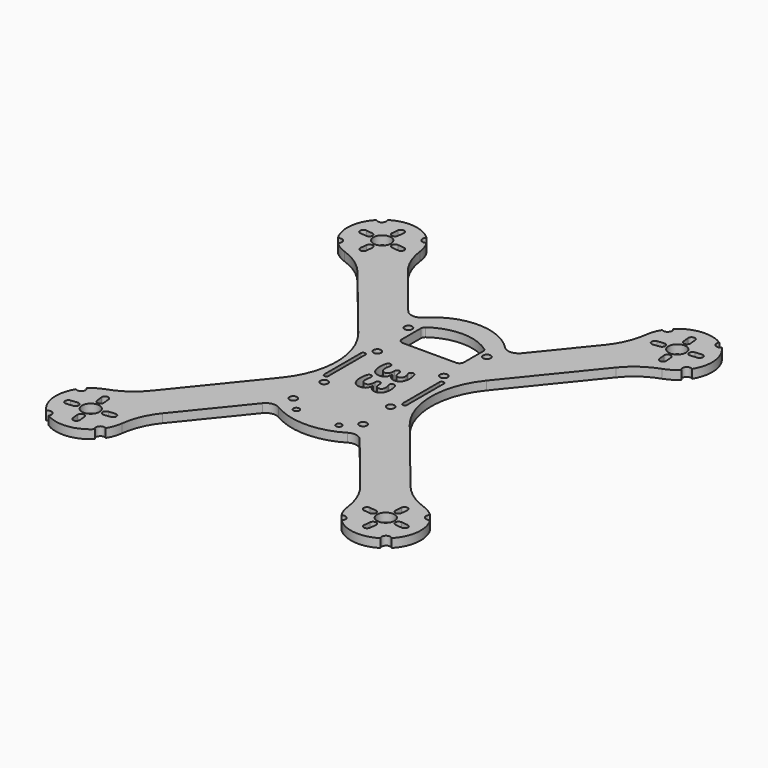
from build123d import *

# Parameters (mm, degrees)
F0_R        = 4
F0_R_2      = 1.35
F0_R_3      = 1.75
F1_DEPTH    = 4
F2_T1_DEPTH = 4


# Not quite as in the source:
# - a fillet or chamfer that OpenCascade refuses, or shapes differently, is made with other operations: its cross-section is extruded or revolved along the edge and cut away or added


with BuildPart() as f1:
    # F0 (on Top) → F1 (new body)
    with BuildSketch(Plane.XY):
        with BuildLine():
            ThreePointArc((59.2954813788, 58.9226797885), (65.4077135301, 64.6212321295), (72.8546961891, 68.4127133611))
            ThreePointArc((72.8546961891, 68.4127133611), (75.9892117021, 69.8870591003), (78.732954082, 72.0014764226))
            ThreePointArc((78.732954082, 72.0014764226), (78.5319854983, 74.7327053819), (81.2453142699, 75.1039828748))
            ThreePointArc((81.2453142699, 75.1039828748), (83.5642923637, 85.2156462689), (79.1936564719, 94.6242029008))
            ThreePointArc((79.1936564719, 94.6242029008), (76.4624275126, 94.423234317), (76.0911500197, 97.1365630887))
            ThreePointArc((76.0911500197, 97.1365630887), (65.9794866256, 99.4555411825), (56.5709299937, 95.0849052907))
            ThreePointArc((56.5709299937, 95.0849052907), (56.7718985775, 92.3536763313), (54.0585698058, 91.9823988384))
            ThreePointArc((54.0585698058, 91.9823988384), (52.5608136924, 88.8590017319), (51.7703883652, 85.4864491879))
            ThreePointArc((51.7703883652, 85.4864491879), (49.6100748513, 77.4139076937), (45.3068540726, 70.2504468274))
            Line((45.3068540726, 70.2504468274), (26.0751424851, 46.5012608726))
            ThreePointArc((26.0751424851, 46.5012608726), (22.420247462, 44.6531941399), (18.6104751491, 46.1562720492))
            ThreePointArc((18.6104751491, 46.1562720492), (0, 54), (-18.6104751491, 46.1562720492))
            ThreePointArc((-18.6104751491, 46.1562720492), (-22.420247462, 44.6531941399), (-26.0751424851, 46.5012608726))
            Line((-26.0751424851, 46.5012608726), (-45.3068540726, 70.2504468274))
            ThreePointArc((-45.3068540726, 70.2504468274), (-49.6100748513, 77.4139076937), (-51.7703883652, 85.4864491879))
            ThreePointArc((-51.7703883652, 85.4864491879), (-52.5608136924, 88.8590017319), (-54.0585698058, 91.9823988384))
            ThreePointArc((-54.0585698058, 91.9823988384), (-56.7718985775, 92.3536763313), (-56.5709299937, 95.0849052907))
            ThreePointArc((-56.5709299937, 95.0849052907), (-65.9794866256, 99.4555411825), (-76.0911500197, 97.1365630887))
            ThreePointArc((-76.0911500197, 97.1365630887), (-76.4624275126, 94.423234317), (-79.1936564719, 94.6242029008))
            ThreePointArc((-79.1936564719, 94.6242029008), (-83.5642923637, 85.2156462689), (-81.2453142699, 75.1039828748))
            ThreePointArc((-81.2453142699, 75.1039828748), (-78.5319854983, 74.7327053819), (-78.732954082, 72.0014764226))
            ThreePointArc((-78.732954082, 72.0014764226), (-75.9892117021, 69.8870591003), (-72.8546961891, 68.4127133611))
            ThreePointArc((-72.8546961891, 68.4127133611), (-65.4077135301, 64.6212321295), (-59.2954813788, 58.9226797885))
            Line((-59.2954813788, 58.9226797885), (-29.4173122483, 22.0262136867))
            ThreePointArc((-29.4173122483, 22.0262136867), (-21.6174208993, 0), (-29.4173122483, -22.0262136867))
            Line((-29.4173122483, -22.0262136867), (-59.2954813788, -58.9226797885))
            ThreePointArc((-59.2954813788, -58.9226797885), (-65.4077135301, -64.6212321295), (-72.8546961891, -68.4127133611))
            ThreePointArc((-72.8546961891, -68.4127133611), (-75.9892117021, -69.8870591003), (-78.732954082, -72.0014764226))
            ThreePointArc((-78.732954082, -72.0014764226), (-78.5319854983, -74.7327053819), (-81.2453142699, -75.1039828748))
            ThreePointArc((-81.2453142699, -75.1039828748), (-83.5642923637, -85.2156462689), (-79.1936564719, -94.6242029008))
            ThreePointArc((-79.1936564719, -94.6242029008), (-76.4624275126, -94.423234317), (-76.0911500197, -97.1365630887))
            ThreePointArc((-76.0911500197, -97.1365630887), (-65.9794866256, -99.4555411825), (-56.5709299937, -95.0849052907))
            ThreePointArc((-56.5709299937, -95.0849052907), (-56.7718985775, -92.3536763313), (-54.0585698058, -91.9823988384))
            ThreePointArc((-54.0585698058, -91.9823988384), (-52.5608136924, -88.8590017319), (-51.7703883652, -85.4864491879))
            ThreePointArc((-51.7703883652, -85.4864491879), (-49.6100748513, -77.4139076937), (-45.3068540726, -70.2504468274))
            Line((-45.3068540726, -70.2504468274), (-22.2716253028, -41.8043083194))
            ThreePointArc((-22.2716253028, -41.8043083194), (-19.2665196055, -40.0290710679), (-15.8322988989, -40.6521727365))
            ThreePointArc((-15.8322988989, -40.6521727365), (0, -45), (15.8322988989, -40.6521727365))
            ThreePointArc((15.8322988989, -40.6521727365), (19.2665196055, -40.0290710679), (22.2716253028, -41.8043083194))
            Line((22.2716253028, -41.8043083194), (45.3068540726, -70.2504468274))
            ThreePointArc((45.3068540726, -70.2504468274), (49.6100748513, -77.4139076937), (51.7703883652, -85.4864491879))
            ThreePointArc((51.7703883652, -85.4864491879), (52.5608136924, -88.8590017319), (54.0585698058, -91.9823988384))
            ThreePointArc((54.0585698058, -91.9823988384), (56.7718985775, -92.3536763313), (56.5709299937, -95.0849052907))
            ThreePointArc((56.5709299937, -95.0849052907), (65.9794866256, -99.4555411825), (76.0911500197, -97.1365630887))
            ThreePointArc((76.0911500197, -97.1365630887), (76.4624275126, -94.423234317), (79.1936564719, -94.6242029008))
            ThreePointArc((79.1936564719, -94.6242029008), (83.5642923637, -85.2156462689), (81.2453142699, -75.1039828748))
            ThreePointArc((81.2453142699, -75.1039828748), (78.5319854983, -74.7327053819), (78.732954082, -72.0014764226))
            ThreePointArc((78.732954082, -72.0014764226), (75.9892117021, -69.8870591003), (72.8546961891, -68.4127133611))
            ThreePointArc((72.8546961891, -68.4127133611), (65.4077135301, -64.6212321295), (59.2954813788, -58.9226797885))
            Line((59.2954813788, -58.9226797885), (29.4173122483, -22.0262136867))
            ThreePointArc((29.4173122483, -22.0262136867), (21.6174208993, 0), (29.4173122483, 22.0262136867))
            Line((29.4173122483, 22.0262136867), (59.2954813788, 58.9226797885))
        make_face()
        with BuildLine():
            Line((-68.1507044799, -93.1479415575), (-68.4642898697, -90.1643758714))
            ThreePointArc((-68.4642898697, -90.1643758714), (-67.1292997215, -88.5158003335), (-65.4807241836, -89.8507904816))
            Line((-65.4807241836, -89.8507904816), (-65.1671387938, -92.8343561677))
            ThreePointArc((-65.1671387938, -92.8343561677), (-66.5021289419, -94.4829317057), (-68.1507044799, -93.1479415575))
        make_face(mode=Mode.SUBTRACT)
        with BuildLine():
            Line((-77.2566927388, -83.0444284146), (-74.2731270527, -82.7308430248))
            ThreePointArc((-74.2731270527, -82.7308430248), (-72.6245515147, -84.065833173), (-73.9595416628, -85.7144087109))
            Line((-73.9595416628, -85.7144087109), (-76.943107349, -86.0279941007))
            ThreePointArc((-76.943107349, -86.0279941007), (-78.5916828869, -84.6930039526), (-77.2566927388, -83.0444284146))
        make_face(mode=Mode.SUBTRACT)
        with Locations((-67.6519420379, -83.5431908566)):
            Circle(F0_R, mode=Mode.SUBTRACT)
        with BuildLine():
            ThreePointArc((-66.839594206, -76.9220058418), (-68.1745843542, -78.5705813798), (-69.8231598921, -77.2355912316))
            Line((-69.8231598921, -77.2355912316), (-70.136745282, -74.2520255455))
            ThreePointArc((-70.136745282, -74.2520255455), (-68.8017551338, -72.6034500076), (-67.1531795958, -73.9384401557))
            Line((-67.1531795958, -73.9384401557), (-66.839594206, -76.9220058418))
        make_face(mode=Mode.SUBTRACT)
        with BuildLine():
            Line((-58.047191337, -84.0419532986), (-61.0307570231, -84.3555386884))
            ThreePointArc((-61.0307570231, -84.3555386884), (-62.679332561, -83.0205485403), (-61.3443424129, -81.3719730023))
            Line((-61.3443424129, -81.3719730023), (-58.3607767268, -81.0583876125))
            ThreePointArc((-58.3607767268, -81.0583876125), (-56.7122011888, -82.3933777607), (-58.047191337, -84.0419532986))
        make_face(mode=Mode.SUBTRACT)
        with Locations((-9.75, -38)):
            Circle(F0_R_2, mode=Mode.SUBTRACT)
        with Locations((-16, -32)):
            Circle(F0_R_3, mode=Mode.SUBTRACT)
        with Locations((-15.25, -15.25)):
            Circle(F0_R_3, mode=Mode.SUBTRACT)
        with BuildLine():
            add(Edge.make_bspline(
                [(6.2055121528, -8.4370659722), (5.33203125, -9.6857638889), (3.7764756944, -9.6857638889)],
                knots=[0, 0, 0, 1, 1, 1], degree=2))
            add(Edge.make_bspline(
                [(3.7764756944, -9.6857638889), (2.4761284722, -9.6857638889), (1.5646701389, -8.8973524306)],
                knots=[0, 0, 0, 1, 1, 1], degree=2))
            add(Edge.make_bspline(
                [(1.5646701389, -8.8973524306), (0.6532118056, -8.1089409722), (0.3098958333, -6.6840277778)],
                knots=[0, 0, 0, 1, 1, 1], degree=2))
            Line((0.3098958333, -6.6840277778), (0.2552083333, -6.6840277778))
            add(Edge.make_bspline(
                [(0.2552083333, -6.6840277778), (0.0455729167, -8.3671875), (-0.7671440972, -9.2300347222)],
                knots=[0, 0, 0, 1, 1, 1], degree=2))
            add(Edge.make_bspline(
                [(-0.7671440972, -9.2300347222), (-1.5798611111, -10.0928819444), (-2.9561631944, -10.0928819444)],
                knots=[0, 0, 0, 1, 1, 1], degree=2))
            add(Edge.make_bspline(
                [(-2.9561631944, -10.0928819444), (-4.9583333333, -10.0928819444), (-6.0748697917, -8.640625)],
                knots=[0, 0, 0, 1, 1, 1], degree=2))
            add(Edge.make_bspline(
                [(-6.0748697917, -8.640625), (-7.19140625, -7.1883680556), (-7.19140625, -4.4934895833)],
                knots=[0, 0, 0, 1, 1, 1], degree=2))
            add(Edge.make_bspline(
                [(-7.19140625, -4.4934895833), (-7.19140625, -2.2330729167), (-6.4409722222, -0.4861111111)],
                knots=[0, 0, 0, 1, 1, 1], degree=2))
            Line((-6.4409722222, -0.4861111111), (-3.9435763889, -0.4861111111))
            add(Edge.make_bspline(
                [(-3.9435763889, -0.4861111111), (-4.3506944444, -1.2912326389), (-4.607421875, -2.2604166667)],
                knots=[0, 0, 0, 1, 1, 1], degree=2))
            add(Edge.make_bspline(
                [(-4.607421875, -2.2604166667), (-4.8641493056, -3.2296006944), (-4.8641493056, -4.1775173611)],
                knots=[0, 0, 0, 1, 1, 1], degree=2))
            add(Edge.make_bspline(
                [(-4.8641493056, -4.1775173611), (-4.8641493056, -5.6328125), (-4.3704427083, -6.3255208333)],
                knots=[0, 0, 0, 1, 1, 1], degree=2))
            add(Edge.make_bspline(
                [(-4.3704427083, -6.3255208333), (-3.8767361111, -7.0182291667), (-2.7829861111, -7.0182291667)],
                knots=[0, 0, 0, 1, 1, 1], degree=2))
            add(Edge.make_bspline(
                [(-2.7829861111, -7.0182291667), (-1.8077256944, -7.0182291667), (-1.3990885417, -6.220703125)],
                knots=[0, 0, 0, 1, 1, 1], degree=2))
            add(Edge.make_bspline(
                [(-1.3990885417, -6.220703125), (-0.9904513889, -5.4231770833), (-0.9904513889, -3.6762152778)],
                knots=[0, 0, 0, 1, 1, 1], degree=2))
            Line((-0.9904513889, -3.6762152778), (-0.9904513889, -2.6219618056))
            Line((-0.9904513889, -2.6219618056), (1.2608506944, -2.6219618056))
            Line((1.2608506944, -2.6219618056), (1.2608506944, -3.6944444444))
            add(Edge.make_bspline(
                [(1.2608506944, -3.6944444444), (1.2608506944, -5.3077256944), (1.6831597222, -6.0536024306)],
                knots=[0, 0, 0, 1, 1, 1], degree=2))
            add(Edge.make_bspline(
                [(1.6831597222, -6.0536024306), (2.10546875, -6.7994791667), (3.1293402778, -6.7994791667)],
                knots=[0, 0, 0, 1, 1, 1], degree=2))
            add(Edge.make_bspline(
                [(3.1293402778, -6.7994791667), (4.7061631944, -6.7994791667), (4.7061631944, -4.8246527778)],
                knots=[0, 0, 0, 1, 1, 1], degree=2))
            add(Edge.make_bspline(
                [(4.7061631944, -4.8246527778), (4.7061631944, -4.1410590278), (4.4782986111, -3.4331597222)],
                knots=[0, 0, 0, 1, 1, 1], degree=2))
            add(Edge.make_bspline(
                [(4.4782986111, -3.4331597222), (4.2504340278, -2.7252604167), (3.69140625, -1.8624131944)],
                knots=[0, 0, 0, 1, 1, 1], degree=2))
            Line((3.69140625, -1.8624131944), (5.7118055556, -0.5043402778))
            add(Edge.make_bspline(
                [(5.7118055556, -0.5043402778), (7.0789930556, -2.4032118056), (7.0789930556, -5.0342881944)],
                knots=[0, 0, 0, 1, 1, 1], degree=2))
            add(Edge.make_bspline(
                [(7.0789930556, -5.0342881944), (7.0789930556, -7.1883680556), (6.2055121528, -8.4370659722)],
                knots=[0, 0, 0, 1, 1, 1], degree=2))
        make_face(mode=Mode.SUBTRACT)
        with BuildLine():
            ThreePointArc((61.3443424129, -81.3719730023), (62.679332561, -83.0205485403), (61.0307570231, -84.3555386884))
            Line((61.0307570231, -84.3555386884), (58.047191337, -84.0419532986))
            ThreePointArc((58.047191337, -84.0419532986), (56.7122011888, -82.3933777607), (58.3607767268, -81.0583876125))
            Line((58.3607767268, -81.0583876125), (61.3443424129, -81.3719730023))
        make_face(mode=Mode.SUBTRACT)
        with BuildLine():
            ThreePointArc((65.4807241836, -89.8507904816), (67.1292997215, -88.5158003335), (68.4642898697, -90.1643758714))
            Line((68.4642898697, -90.1643758714), (68.1507044799, -93.1479415575))
            ThreePointArc((68.1507044799, -93.1479415575), (66.5021289419, -94.4829317057), (65.1671387938, -92.8343561677))
            Line((65.1671387938, -92.8343561677), (65.4807241836, -89.8507904816))
        make_face(mode=Mode.SUBTRACT)
        with Locations((67.6519420379, -83.5431908566)):
            Circle(F0_R, mode=Mode.SUBTRACT)
        with BuildLine():
            ThreePointArc((69.8231598921, -77.2355912316), (68.1745843542, -78.5705813798), (66.839594206, -76.9220058418))
            Line((66.839594206, -76.9220058418), (67.1531795958, -73.9384401557))
            ThreePointArc((67.1531795958, -73.9384401557), (68.8017551338, -72.6034500076), (70.136745282, -74.2520255455))
            Line((70.136745282, -74.2520255455), (69.8231598921, -77.2355912316))
        make_face(mode=Mode.SUBTRACT)
        with BuildLine():
            ThreePointArc((73.9595416628, -85.7144087109), (72.6245515147, -84.065833173), (74.2731270527, -82.7308430248))
            Line((74.2731270527, -82.7308430248), (77.2566927388, -83.0444284146))
            ThreePointArc((77.2566927388, -83.0444284146), (78.5916828869, -84.6930039526), (76.943107349, -86.0279941007))
            Line((76.943107349, -86.0279941007), (73.9595416628, -85.7144087109))
        make_face(mode=Mode.SUBTRACT)
        with Locations((9.75, -38)):
            Circle(F0_R_2, mode=Mode.SUBTRACT)
        with Locations((16, -32)):
            Circle(F0_R_3, mode=Mode.SUBTRACT)
        with Locations((15.25, -15.25)):
            Circle(F0_R_3, mode=Mode.SUBTRACT)
        with BuildLine():
            Line((-19, -10.5), (-19, 10.5))
            ThreePointArc((-19, 10.5), (-18, 11.5), (-17, 10.5))
            Line((-17, 10.5), (-17, -10.5))
            ThreePointArc((-17, -10.5), (-18, -11.5), (-19, -10.5))
        make_face(mode=Mode.SUBTRACT)
        with BuildLine():
            add(Edge.make_bspline(
                [(6.2055121528, 2.6614583333), (5.33203125, 1.4127604167), (3.7764756944, 1.4127604167)],
                knots=[0, 0, 0, 1, 1, 1], degree=2))
            add(Edge.make_bspline(
                [(3.7764756944, 1.4127604167), (2.4761284722, 1.4127604167), (1.5646701389, 2.201171875)],
                knots=[0, 0, 0, 1, 1, 1], degree=2))
            add(Edge.make_bspline(
                [(1.5646701389, 2.201171875), (0.6532118056, 2.9895833333), (0.3098958333, 4.4144965278)],
                knots=[0, 0, 0, 1, 1, 1], degree=2))
            Line((0.3098958333, 4.4144965278), (0.2552083333, 4.4144965278))
            add(Edge.make_bspline(
                [(0.2552083333, 4.4144965278), (0.0455729167, 2.7313368056), (-0.7671440972, 1.8684895833)],
                knots=[0, 0, 0, 1, 1, 1], degree=2))
            add(Edge.make_bspline(
                [(-0.7671440972, 1.8684895833), (-1.5798611111, 1.0056423611), (-2.9561631944, 1.0056423611)],
                knots=[0, 0, 0, 1, 1, 1], degree=2))
            add(Edge.make_bspline(
                [(-2.9561631944, 1.0056423611), (-4.9583333333, 1.0056423611), (-6.0748697917, 2.4578993056)],
                knots=[0, 0, 0, 1, 1, 1], degree=2))
            add(Edge.make_bspline(
                [(-6.0748697917, 2.4578993056), (-7.19140625, 3.91015625), (-7.19140625, 6.6050347222)],
                knots=[0, 0, 0, 1, 1, 1], degree=2))
            add(Edge.make_bspline(
                [(-7.19140625, 6.6050347222), (-7.19140625, 8.8654513889), (-6.4409722222, 10.6124131944)],
                knots=[0, 0, 0, 1, 1, 1], degree=2))
            Line((-6.4409722222, 10.6124131944), (-3.9435763889, 10.6124131944))
            add(Edge.make_bspline(
                [(-3.9435763889, 10.6124131944), (-4.3506944444, 9.8072916667), (-4.607421875, 8.8381076389)],
                knots=[0, 0, 0, 1, 1, 1], degree=2))
            add(Edge.make_bspline(
                [(-4.607421875, 8.8381076389), (-4.8641493056, 7.8689236111), (-4.8641493056, 6.9210069444)],
                knots=[0, 0, 0, 1, 1, 1], degree=2))
            add(Edge.make_bspline(
                [(-4.8641493056, 6.9210069444), (-4.8641493056, 5.4657118056), (-4.3704427083, 4.7730034722)],
                knots=[0, 0, 0, 1, 1, 1], degree=2))
            add(Edge.make_bspline(
                [(-4.3704427083, 4.7730034722), (-3.8767361111, 4.0802951389), (-2.7829861111, 4.0802951389)],
                knots=[0, 0, 0, 1, 1, 1], degree=2))
            add(Edge.make_bspline(
                [(-2.7829861111, 4.0802951389), (-1.8077256944, 4.0802951389), (-1.3990885417, 4.8778211806)],
                knots=[0, 0, 0, 1, 1, 1], degree=2))
            add(Edge.make_bspline(
                [(-1.3990885417, 4.8778211806), (-0.9904513889, 5.6753472222), (-0.9904513889, 7.4223090278)],
                knots=[0, 0, 0, 1, 1, 1], degree=2))
            Line((-0.9904513889, 7.4223090278), (-0.9904513889, 8.4765625))
            Line((-0.9904513889, 8.4765625), (1.2608506944, 8.4765625))
            Line((1.2608506944, 8.4765625), (1.2608506944, 7.4040798611))
            add(Edge.make_bspline(
                [(1.2608506944, 7.4040798611), (1.2608506944, 5.7907986111), (1.6831597222, 5.044921875)],
                knots=[0, 0, 0, 1, 1, 1], degree=2))
            add(Edge.make_bspline(
                [(1.6831597222, 5.044921875), (2.10546875, 4.2990451389), (3.1293402778, 4.2990451389)],
                knots=[0, 0, 0, 1, 1, 1], degree=2))
            add(Edge.make_bspline(
                [(3.1293402778, 4.2990451389), (4.7061631944, 4.2990451389), (4.7061631944, 6.2738715278)],
                knots=[0, 0, 0, 1, 1, 1], degree=2))
            add(Edge.make_bspline(
                [(4.7061631944, 6.2738715278), (4.7061631944, 6.9574652778), (4.4782986111, 7.6653645833)],
                knots=[0, 0, 0, 1, 1, 1], degree=2))
            add(Edge.make_bspline(
                [(4.4782986111, 7.6653645833), (4.2504340278, 8.3732638889), (3.69140625, 9.2361111111)],
                knots=[0, 0, 0, 1, 1, 1], degree=2))
            Line((3.69140625, 9.2361111111), (5.7118055556, 10.5941840278))
            add(Edge.make_bspline(
                [(5.7118055556, 10.5941840278), (7.0789930556, 8.6953125), (7.0789930556, 6.0642361111)],
                knots=[0, 0, 0, 1, 1, 1], degree=2))
            add(Edge.make_bspline(
                [(7.0789930556, 6.0642361111), (7.0789930556, 3.91015625), (6.2055121528, 2.6614583333)],
                knots=[0, 0, 0, 1, 1, 1], degree=2))
        make_face(mode=Mode.SUBTRACT)
        with Locations((-15.25, 15.25)):
            Circle(F0_R_3, mode=Mode.SUBTRACT)
        with Locations((-18, 36.5)):
            Circle(F0_R_3, mode=Mode.SUBTRACT)
        with BuildLine():
            ThreePointArc((-73.9595416628, 85.7144087109), (-72.6245515147, 84.065833173), (-74.2731270527, 82.7308430248))
            Line((-74.2731270527, 82.7308430248), (-77.2566927388, 83.0444284146))
            ThreePointArc((-77.2566927388, 83.0444284146), (-78.5916828869, 84.6930039526), (-76.943107349, 86.0279941007))
            Line((-76.943107349, 86.0279941007), (-73.9595416628, 85.7144087109))
        make_face(mode=Mode.SUBTRACT)
        with BuildLine():
            ThreePointArc((-69.8231598921, 77.2355912316), (-68.1745843542, 78.5705813798), (-66.839594206, 76.9220058418))
            Line((-66.839594206, 76.9220058418), (-67.1531795958, 73.9384401557))
            ThreePointArc((-67.1531795958, 73.9384401557), (-68.8017551338, 72.6034500076), (-70.136745282, 74.2520255455))
            Line((-70.136745282, 74.2520255455), (-69.8231598921, 77.2355912316))
        make_face(mode=Mode.SUBTRACT)
        with Locations((-67.6519420379, 83.5431908566)):
            Circle(F0_R, mode=Mode.SUBTRACT)
        with BuildLine():
            ThreePointArc((-65.4807241836, 89.8507904816), (-67.1292997215, 88.5158003335), (-68.4642898697, 90.1643758714))
            Line((-68.4642898697, 90.1643758714), (-68.1507044799, 93.1479415575))
            ThreePointArc((-68.1507044799, 93.1479415575), (-66.5021289419, 94.4829317057), (-65.1671387938, 92.8343561677))
            Line((-65.1671387938, 92.8343561677), (-65.4807241836, 89.8507904816))
        make_face(mode=Mode.SUBTRACT)
        with BuildLine():
            ThreePointArc((-61.3443424129, 81.3719730023), (-62.679332561, 83.0205485403), (-61.0307570231, 84.3555386884))
            Line((-61.0307570231, 84.3555386884), (-58.047191337, 84.0419532986))
            ThreePointArc((-58.047191337, 84.0419532986), (-56.7122011888, 82.3933777607), (-58.3607767268, 81.0583876125))
            Line((-58.3607767268, 81.0583876125), (-61.3443424129, 81.3719730023))
        make_face(mode=Mode.SUBTRACT)
        with BuildLine():
            Line((19, 10.5), (19, -10.5))
            ThreePointArc((19, -10.5), (18, -11.5), (17, -10.5))
            Line((17, -10.5), (17, 10.5))
            ThreePointArc((17, 10.5), (18, 11.5), (19, 10.5))
        make_face(mode=Mode.SUBTRACT)
        with Locations((15.25, 15.25)):
            Circle(F0_R_3, mode=Mode.SUBTRACT)
        with BuildLine():
            Line((12.25, 26), (-12.25, 26))
            ThreePointArc((-12.25, 26), (-13.6642135624, 26.5857864376), (-14.25, 28))
            Line((-14.25, 28), (-14.25, 39.0031508785))
            ThreePointArc((-14.25, 39.0031508785), (-14.029513042, 39.9160218077), (-13.4166666667, 40.6276166027))
            ThreePointArc((-13.4166666667, 40.6276166027), (0, 44.9462607751), (13.4166666667, 40.6276166027))
            ThreePointArc((13.4166666667, 40.6276166027), (14.029513042, 39.9160218077), (14.25, 39.0031508785))
            Line((14.25, 39.0031508785), (14.25, 28))
            ThreePointArc((14.25, 28), (13.6642135624, 26.5857864376), (12.25, 26))
        make_face(mode=Mode.SUBTRACT)
        with Locations((18, 36.5)):
            Circle(F0_R_3, mode=Mode.SUBTRACT)
        with BuildLine():
            Line((61.3443424129, 81.3719730023), (58.3607767268, 81.0583876125))
            ThreePointArc((58.3607767268, 81.0583876125), (56.7122011888, 82.3933777607), (58.047191337, 84.0419532986))
            Line((58.047191337, 84.0419532986), (61.0307570231, 84.3555386884))
            ThreePointArc((61.0307570231, 84.3555386884), (62.679332561, 83.0205485403), (61.3443424129, 81.3719730023))
        make_face(mode=Mode.SUBTRACT)
        with BuildLine():
            ThreePointArc((66.839594206, 76.9220058418), (68.1745843542, 78.5705813798), (69.8231598921, 77.2355912316))
            Line((69.8231598922, 77.2355912316), (70.136745282, 74.2520255455))
            ThreePointArc((70.136745282, 74.2520255455), (68.8017551338, 72.6034500076), (67.1531795958, 73.9384401557))
            Line((67.1531795958, 73.9384401557), (66.839594206, 76.9220058418))
        make_face(mode=Mode.SUBTRACT)
        with Locations((67.6519420379, 83.5431908566)):
            Circle(F0_R, mode=Mode.SUBTRACT)
        with BuildLine():
            Line((77.2566927388, 83.0444284146), (74.2731270527, 82.7308430248))
            ThreePointArc((74.2731270527, 82.7308430248), (72.6245515147, 84.065833173), (73.9595416628, 85.7144087109))
            Line((73.9595416628, 85.7144087109), (76.943107349, 86.0279941007))
            ThreePointArc((76.943107349, 86.0279941007), (78.5916828869, 84.6930039526), (77.2566927388, 83.0444284146))
        make_face(mode=Mode.SUBTRACT)
        with BuildLine():
            ThreePointArc((68.4642898697, 90.1643758714), (67.1292997215, 88.5158003335), (65.4807241836, 89.8507904816))
            Line((65.4807241836, 89.8507904816), (65.1671387938, 92.8343561677))
            ThreePointArc((65.1671387938, 92.8343561677), (66.5021289419, 94.4829317057), (68.1507044799, 93.1479415575))
            Line((68.1507044799, 93.1479415575), (68.4642898697, 90.1643758714))
        make_face(mode=Mode.SUBTRACT)
    extrude(amount=F1_DEPTH)

    # F2: fillet of radius 1.2 on 12 edges, made by hand

    # F2_s2 → F2_t1 (join)
    with BuildSketch(Plane.XY):
        with BuildLine():
            ThreePointArc((-6.7524030076, 9.7637954228), (-6.3175481088, 10.3775410431), (-5.60310463, 10.6128131944))
            Line((-5.60310463, 10.6128131944), (-5.60310463, 10.7330531944))
            ThreePointArc((-5.60310463, 10.7330531944), (-6.0220384261, 10.7326531944), (-6.4409722222, 10.7326531944))
            Line((-6.4409722222, 10.7326531944), (-6.5514504294, 10.6598707895))
            ThreePointArc((-6.5514504294, 10.6598707895), (-6.7208196841, 10.2335448862), (-6.8673328453, 9.7991336456))
            Line((-6.8673328453, 9.7991336456), (-6.7524030076, 9.7637954228))
        make_face()
        with BuildLine():
            ThreePointArc((-5.6938913584, 10.6128131944), (-4.733651679, 10.1330532603), (-4.5406824541, 9.077121106))
            Line((-4.5406824541, 9.077121106), (-4.4253615637, 9.0436358969))
            ThreePointArc((-4.4253615637, 9.0436358969), (-4.1659655391, 9.8153107066), (-3.836413723, 10.5582252804))
            Line((-3.836413723, 10.5582252804), (-3.9435763889, 10.7324971942))
            ThreePointArc((-3.9435763889, 10.7324971942), (-4.8187338736, 10.7324971942), (-5.6938913584, 10.7328971942))
            Line((-5.6938913584, 10.7328971942), (-5.6938913584, 10.6128131944))
        make_face()
        with BuildLine():
            ThreePointArc((-0.9914789372, 7.2868485876), (-0.6356723059, 8.1290594687), (0.209834056, 8.4769625))
            Line((0.209834056, 8.4769625), (0.209834056, 8.5970990685))
            ThreePointArc((0.209834056, 8.5970990685), (-0.3903086664, 8.5966990685), (-0.9904513889, 8.5966990685))
            Line((-0.9904513889, 8.5966990685), (-1.1105879574, 8.4765625))
            ThreePointArc((-1.1105879574, 8.4765625), (-1.1105879574, 7.4223090278), (-1.1116102365, 7.2879737649))
            Line((-1.1116102365, 7.2879737649), (-0.9914789372, 7.2868485876))
        make_face()
        with BuildLine():
            ThreePointArc((0.0605062724, 8.4769625), (0.9058451255, 8.1292253835), (1.2618147568, 7.2873201037))
            Line((1.2618147568, 7.2873201037), (1.3819456052, 7.2884924326))
            ThreePointArc((1.3819456052, 7.2884924326), (1.380987263, 7.4040798611), (1.380987263, 8.4765625))
            Line((1.380987263, 8.4765625), (1.2608506944, 8.5966990685))
            ThreePointArc((1.2608506944, 8.5966990685), (0.6606784834, 8.5966990685), (0.0605062724, 8.5970990685))
            Line((0.0605062724, 8.5970990685), (0.0605062724, 8.4769625))
        make_face()
        with BuildLine():
            ThreePointArc((4.204619479, 8.3361108824), (4.1256243356, 9.173607687), (4.6152952395, 9.857613196))
            Line((4.6152952395, 9.857613196), (4.5482737644, 9.9573207596))
            ThreePointArc((4.5482737644, 9.9573207596), (4.0864408425, 9.6464037307), (3.6243847749, 9.3358186748))
            Line((3.6243847749, 9.3358186748), (3.5905789093, 9.1707863551))
            ThreePointArc((3.5905789093, 9.1707863551), (3.8577235407, 8.7342614728), (4.0965304278, 8.2836682147))
            Line((4.0965304278, 8.2836682147), (4.204619479, 8.3361108824))
        make_face()
        with BuildLine():
            ThreePointArc((4.6493321941, 9.8804921715), (5.6497294573, 10.0385570957), (6.4154886357, 9.3756905291))
            Line((6.4154886357, 9.3756905291), (6.5250813302, 9.4249201223))
            ThreePointArc((6.5250813302, 9.4249201223), (6.1983681216, 10.0627170753), (5.8093049528, 10.6643835938))
            Line((5.8093049528, 10.6643835938), (5.6447826058, 10.6938937852))
            ThreePointArc((5.6447826058, 10.6938937852), (5.113657498, 10.3368818706), (4.5823092444, 9.9802019289))
            Line((4.5823092444, 9.9802019289), (4.6493321941, 9.8804921715))
        make_face()
        with BuildLine():
            ThreePointArc((-6.7524030076, -1.3347288828), (-6.3175481088, -0.7209832624), (-5.60310463, -0.4857111111))
            Line((-5.60310463, -0.4857111111), (-5.60310463, -0.3654711111))
            ThreePointArc((-5.60310463, -0.3654711111), (-6.0220384261, -0.3658711111), (-6.4409722222, -0.3658711111))
            Line((-6.4409722222, -0.3658711111), (-6.5514504294, -0.438653516))
            ThreePointArc((-6.5514504294, -0.438653516), (-6.7208196841, -0.8649794194), (-6.8673328453, -1.29939066))
            Line((-6.8673328453, -1.29939066), (-6.7524030076, -1.3347288828))
        make_face()
        with BuildLine():
            ThreePointArc((-5.6938913584, -0.4857111111), (-4.733651679, -0.9654710453), (-4.5406824541, -2.0214031996))
            Line((-4.5406824541, -2.0214031996), (-4.4253615637, -2.0548884087))
            ThreePointArc((-4.4253615637, -2.0548884087), (-4.1659655391, -1.283213599), (-3.836413723, -0.5402990252))
            Line((-3.836413723, -0.5402990252), (-3.9435763889, -0.3660271114))
            ThreePointArc((-3.9435763889, -0.3660271114), (-4.8187338736, -0.3660271114), (-5.6938913584, -0.3656271114))
            Line((-5.6938913584, -0.3656271114), (-5.6938913584, -0.4857111111))
        make_face()
        with BuildLine():
            ThreePointArc((-0.9914789372, -3.811675718), (-0.6356723059, -2.9694648368), (0.209834056, -2.6215618056))
            Line((0.209834056, -2.6215618056), (0.209834056, -2.501425237))
            ThreePointArc((0.209834056, -2.501425237), (-0.3903086664, -2.501825237), (-0.9904513889, -2.501825237))
            Line((-0.9904513889, -2.501825237), (-1.1105879574, -2.6219618056))
            ThreePointArc((-1.1105879574, -2.6219618056), (-1.1105879574, -3.6762152778), (-1.1116102365, -3.8105505407))
            Line((-1.1116102365, -3.8105505407), (-0.9914789372, -3.811675718))
        make_face()
        with BuildLine():
            ThreePointArc((0.0605062724, -2.6215618056), (0.9058451255, -2.969298922), (1.2618147568, -3.8112042019))
            Line((1.2618147568, -3.8112042019), (1.3819456052, -3.8100318729))
            ThreePointArc((1.3819456052, -3.8100318729), (1.380987263, -3.6944444444), (1.380987263, -2.6219618056))
            Line((1.380987263, -2.6219618056), (1.2608506944, -2.501825237))
            ThreePointArc((1.2608506944, -2.501825237), (0.6606784834, -2.501825237), (0.0605062724, -2.501425237))
            Line((0.0605062724, -2.501425237), (0.0605062724, -2.6215618056))
        make_face()
        with BuildLine():
            ThreePointArc((4.204619479, -2.7624134231), (4.1256243356, -1.9249166185), (4.6152952395, -1.2409111096))
            Line((4.6152952395, -1.2409111096), (4.5482737644, -1.1412035459))
            ThreePointArc((4.5482737644, -1.1412035459), (4.0864408425, -1.4521205748), (3.6243847749, -1.7627056308))
            Line((3.6243847749, -1.7627056308), (3.5905789093, -1.9277379504))
            ThreePointArc((3.5905789093, -1.9277379504), (3.8577235407, -2.3642628327), (4.0965304278, -2.8148560908))
            Line((4.0965304278, -2.8148560908), (4.204619479, -2.7624134231))
        make_face()
        with BuildLine():
            ThreePointArc((6.4154886357, -1.7228337765), (5.6497294573, -1.0599672098), (4.6493321941, -1.2180321341))
            Line((4.6493321941, -1.2180321341), (4.5823092444, -1.1183223767))
            ThreePointArc((4.5823092444, -1.1183223767), (5.113657498, -0.761642435), (5.6447826058, -0.4046305203))
            Line((5.6447826058, -0.4046305203), (5.8093049528, -0.4341407118))
            ThreePointArc((5.8093049528, -0.4341407118), (6.1983681216, -1.0358072303), (6.5250813302, -1.6736041833))
            Line((6.5250813302, -1.6736041833), (6.4154886357, -1.7228337765))
        make_face()
    extrude(amount=F2_T1_DEPTH)


solid = f1.part
